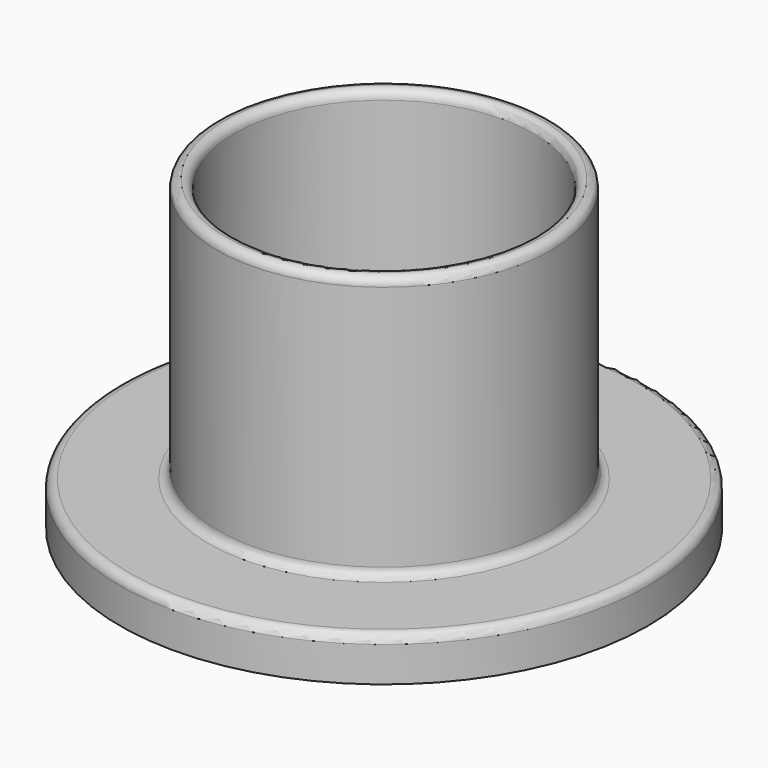
from build123d import *

# Parameters (mm, degrees)
F0_R     = 38.1
F1_DEPTH = 6.35
F2_R     = 24.13
F2_R_2   = 21.59
F3_DEPTH = 38.1
F4_R     = 1.26999


# Not quite as in the source:
# - a fillet or chamfer is up to 0.001 mm smaller than in the source, because OpenCascade refuses the exact size


with BuildPart() as f1:
    # F0 (on Top) → F1 (new body)
    with BuildSketch(Plane.XY):
        Circle(F0_R)
    extrude(amount=F1_DEPTH)

    # F2 (on face) → F3 (join)
    with BuildSketch(Plane.XY.offset(6.35)):
        Circle(F2_R)
        Circle(F2_R_2, mode=Mode.SUBTRACT)
    extrude(amount=F3_DEPTH)

    # F4 (radius 1.27 in the source; OpenCascade refuses exactly that, so slightly less here)
    f4_edges = [f1.edges().sort_by_distance(p)[0] for p in [
        (-21.59, 0, 6.35),
        (-24.13, 0, 6.35),
        (-38.1, 0, 6.35),
        (-21.59, 0, 44.45),
        (-24.13, 0, 44.45),
    ]]
    fillet(f4_edges, radius=F4_R)


solid = f1.part
